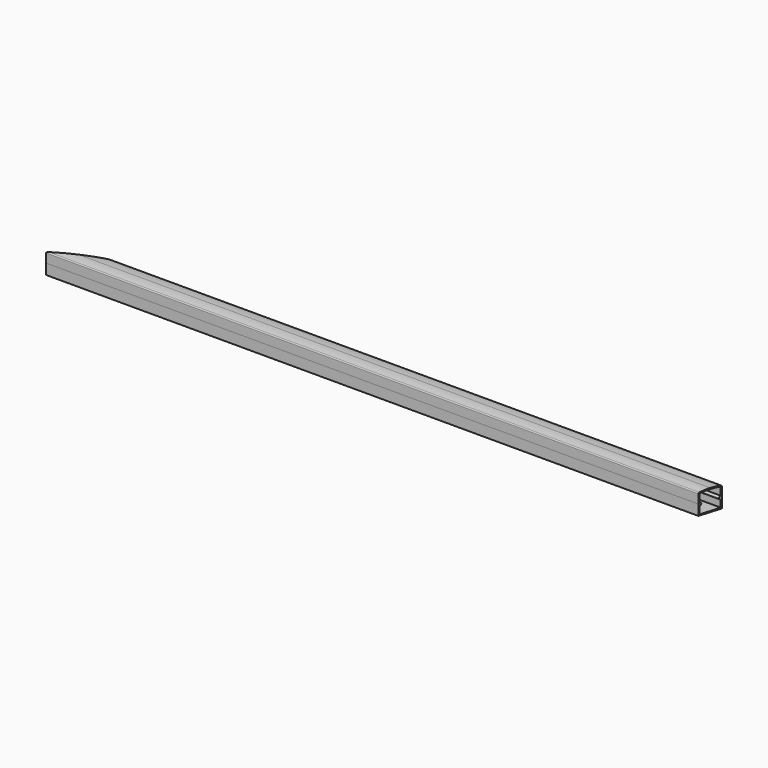
from build123d import *

# Parameters (mm, degrees)
F2_DEPTH      = 1200
F4_DEPTH      = 1200
F8_DEPTH      = 10.001
F8_DEPTH_BACK = 10.001


with BuildPart() as f2:
    # F1 (on Right) → F2 (new body)
    with BuildSketch(Plane.YZ):
        with BuildLine():
            Line((0, -9), (0, -10))
            Line((0, -10), (10, -10))
            Line((10, -10), (10, -0.2))
            Line((10, -0.2), (9, -0.2))
            ThreePointArc((9, -0.2), (8.5, -0.7), (9, -1.2))
            ThreePointArc((9, -1.2), (9.5, -1.7), (9, -2.2))
            Line((9, -2.2), (9, -9))
            Line((9, -9), (0, -9))
        make_face()
    extrude(amount=F2_DEPTH)

    # F5: F2 across plane


with BuildPart() as f4:
    # F3 (on Right) → F4 (new body)
    with BuildSketch(Plane.YZ):
        with BuildLine():
            Line((9, -0.2), (10, -0.2))
            Line((10, -0.2), (10, 8.1663783152))
            ThreePointArc((10, 8.1663783152), (9.7693092582, 8.8052548802), (9.1836734694, 9.1493656277))
            ThreePointArc((9.1836734694, 9.1493656277), (4.6114920912, 9.7868872364), (0, 10))
            Line((0, 10), (0, 9))
            ThreePointArc((0, 9), (4.5192622493, 8.7911494917), (9, 8.1663783152))
            Line((9, 8.1663783152), (9, 0.8))
            ThreePointArc((9, 0.8), (7.5, -0.7), (9, -2.2))
            ThreePointArc((9, -2.2), (9.5, -1.7), (9, -1.2))
            ThreePointArc((9, -1.2), (8.5, -0.7), (9, -0.2))
        make_face()
    extrude(amount=F4_DEPTH)

    # F6: F4 across plane


with BuildPart() as f2_1:
    add(f2.part)
    add(f2.part.mirror(Plane.XZ))


with BuildPart() as f4_1:
    add(f4.part)
    add(f4.part.mirror(Plane.XZ))


with BuildPart() as f8_tool:
    # F7 (on Top) → F8 (new body, two sides)
    with BuildSketch(Plane.XY) as f8_sk:
        Polygon((0, 10), (0, 0), (0, -10), (44.5020182264, 10), align=None)
        Polygon((616.0383560074, 10), (610, -10), (1208.0904245377, -10), (1208.0904245377, 10), align=None)
    extrude(amount=F8_DEPTH)
    extrude(f8_sk.sketch, amount=-F8_DEPTH_BACK)


with BuildPart() as f2_2:
    add(f2_1.part)

    # F8: cut by f8_tool
    add(f8_tool.part, mode=Mode.SUBTRACT)


with BuildPart() as f4_2:
    add(f4_1.part)

    # F8: cut by f8_tool
    add(f8_tool.part, mode=Mode.SUBTRACT)


solid = Compound([f2_2.part, f4_2.part])
